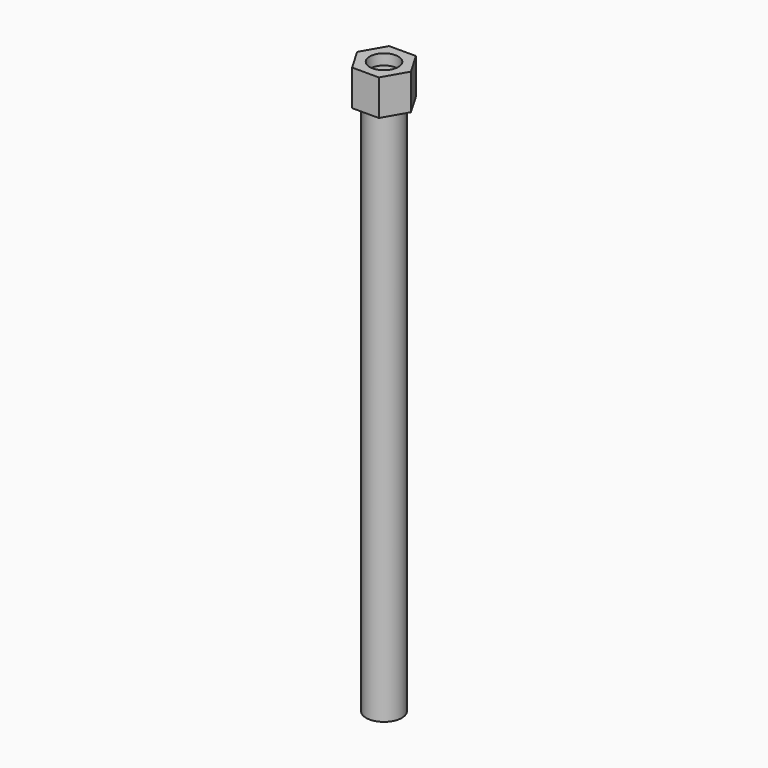
from build123d import *

# Parameters (mm, degrees)
F0_W     = 0.5
F0_H     = 15
F2_R     = 0.5
F3_DEPTH = 1
F4_R     = 0.4
F5_DEPTH = 0.3


with BuildPart() as f1:
    # F0 (on Front) → F1 (revolve)
    with BuildSketch(Plane.XZ):
        with Locations((0.25, 7.5)):
            Rectangle(F0_W, F0_H)
    revolve(axis=Axis((0, 0, 7.5), (0, 0, 1)))

    # F2 (on face) → F3 (join)
    with BuildSketch(Plane.XY.offset(15)):
        Polygon((0.75, 0.0006401425), (0.3744456203, 0.6498391241), (-0.3755543797, 0.6491989816), (-0.75, -0.0006401425), (-0.3744456203, -0.6498391241), (0.3755543797, -0.6491989816), align=None)
        Circle(F2_R, mode=Mode.SUBTRACT)
        Circle(F2_R)
    extrude(amount=F3_DEPTH)

    # F4 (on face) → F5 (cut)
    with BuildSketch(Plane.XY.offset(16)):
        Circle(F4_R)
    extrude(amount=-F5_DEPTH, mode=Mode.SUBTRACT)


solid = f1.part
